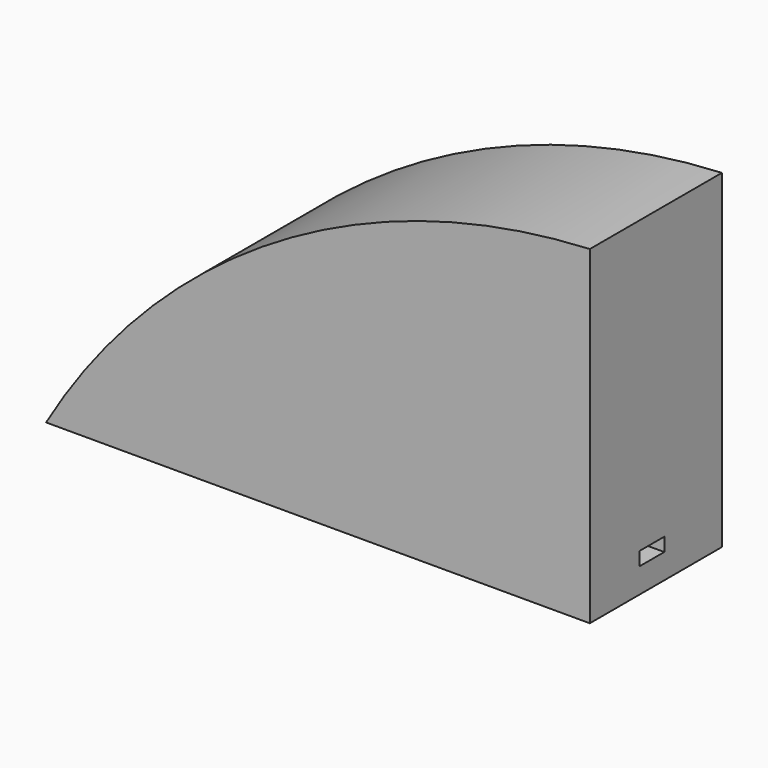
from build123d import *

# Parameters (mm, degrees)
F0_W        = 148.189663887
F0_H        = 89.999999851
F1_DEPTH    = 45
F2_T1_DEPTH = 829.5739384699
F3_W        = 65.8340826631
F3_H        = 55.6846577674
F4_DEPTH    = 25
F5_R        = 10.1457152629
F6_DEPTH    = 22.7
F7_R        = 4.8284271247
F8_W        = 8.5035674274
F8_H        = 3.6853440106
F9_DEPTH    = 58


# Not quite as in the source:
# - a fillet or chamfer that OpenCascade refuses, or shapes differently, is made with other operations: its cross-section is extruded or revolved along the edge and cut away or added


with BuildPart() as f1:
    # F0 (on Front) → F1 (new body)
    with BuildSketch(Plane.XZ):
        with Locations((-0.8728429675, -0.096982345)):
            Rectangle(F0_W, F0_H)
    extrude(amount=F1_DEPTH)

    # F2: fillet of radius 181.7902812467 on 1 edges, made by hand

    # F2_s2 → F2_t1 (cut)
    with BuildSketch(Plane.XZ.offset(-392.286969235)):
        with BuildLine():
            ThreePointArc((81.947112783, 44.9030175805), (-8.4993500697, 20.8059312193), (-74.967674911, -45.0969822705))
            Line((-74.967674911, -45.0969822705), (-74.967674911, 44.9030175805))
            Line((-74.967674911, 44.9030175805), (81.947112783, 44.9030175805))
        make_face()
    extrude(amount=F2_T1_DEPTH, mode=Mode.SUBTRACT)

    # F3 (on face) → F4 (cut)
    with BuildSketch(Plane(origin=(0, 0, 0), x_dir=(-1, 0, 0), z_dir=(0, 1, 0))):
        with Locations((-32.9170413315, -10.9723461792)):
            Rectangle(F3_W, F3_H)
    extrude(amount=-F4_DEPTH, mode=Mode.SUBTRACT)

    # F8 (on face) → F9 (cut)
    with BuildSketch(Plane.YZ.offset(73.221988976)):
        with Locations((-23.8832868636, -36.4655200392)):
            Rectangle(F8_W, F8_H)
    extrude(amount=-F9_DEPTH, mode=Mode.SUBTRACT)


with BuildPart() as f6:
    # F5 (on face) → F6 (new body)
    with BuildSketch(Plane(origin=(0, 0, 0), x_dir=(-1, 0, 0), z_dir=(0, 1, 0))):
        with Locations((-41.4116419852, -25.3735482693)):
            Circle(F5_R)
    extrude(amount=-F6_DEPTH)

    # F7
    f7_edges = [f6.edges().sort_by_distance(p)[0] for p in [
        (51.557357, 0, -25.373548),
    ]]
    fillet(f7_edges, radius=F7_R)


solid = Compound([f1.part, f6.part])
